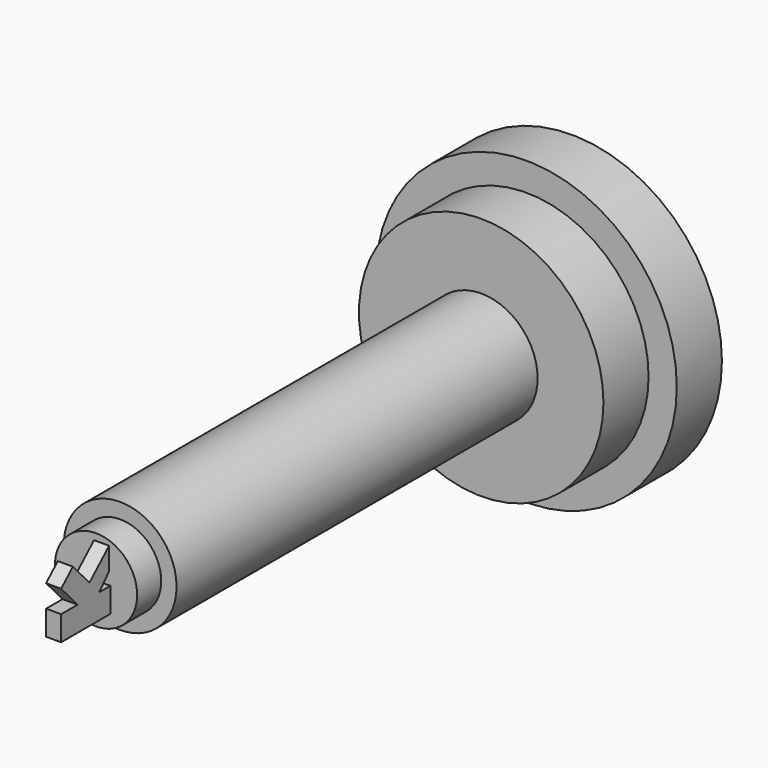
from build123d import *

# Parameters (mm, degrees)
F0_R      = 10.16
F1_DEPTH  = 3.81
F2_R      = 8.255
F3_DEPTH  = 7.62
F4_R      = 3.81
F5_DEPTH  = 38.1
F6_R      = 2.7735730364
F7_DEPTH  = 6.35
F8_DEPTH  = 40.132
F12_DEPTH = 1.016


# Not quite as in the source:
# - a feature names something its author has since deleted; it is built from what else it names
# - the program builds the solid bodies; features that only make, move or delete a surface that nothing else refers to are left out


with BuildPart() as f1:
    # F0 (on Front) → F1 (new body)
    with BuildSketch(Plane.XZ):
        Circle(F0_R)
    extrude(amount=F1_DEPTH)


with BuildPart() as f3:
    # F2 (on Front) → F3 (new body)
    with BuildSketch(Plane.XZ):
        Circle(F2_R)
    extrude(amount=F3_DEPTH)


with BuildPart() as f5:
    # F4 (on Front) → F5 (new body)
    with BuildSketch(Plane.XZ):
        Circle(F4_R)
    extrude(amount=F5_DEPTH)


with BuildPart() as f7:
    # F6 (on Front) → F7 (new body)
    with BuildSketch(Plane.XZ):
        Circle(F6_R)
    extrude(amount=F7_DEPTH)


with BuildPart() as f8:
    # F6 (on Front) → F8 (new body)
    with BuildSketch(Plane.XZ):
        Circle(F6_R)
    extrude(amount=F8_DEPTH)


with BuildPart() as f12:
    # F11 (on Right) → F12 (new body)
    with BuildSketch(Plane.YZ):
        Polygon((-40.1932299137, -1.6699645203), (-40.1932299137, 0), (-41.132259817, 0), (-40.3038863301, 0.9020843856), (-40.3038863301, 2.4242700788), (-41.9606333038, 0.9020843856), (-43.3591868075, 2.4242700788), (-44.350001961, 1.5139291063), (-42.9590344429, 0), (-44.350001961, 0), (-44.350001961, -1.6699645203), align=None)
    extrude(amount=F12_DEPTH)


solid = Compound([f1.part, f3.part, f5.part, f7.part, f8.part, f12.part])
